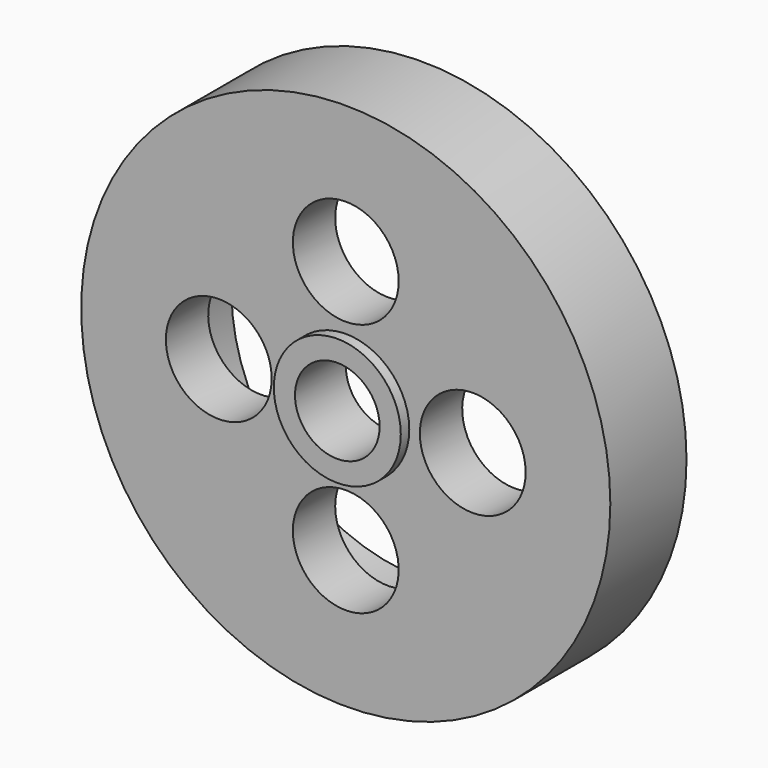
from build123d import *

# Parameters (mm, degrees)
F0_R            = 25
F0_R_2          = 18
F0_R_3          = 6
F0_R_4          = 5
F0_R_5          = 4
F1_DEPTH        = 9
F2_DEPTH        = 10
F3_DEPTH        = 4
F4_DEPTH        = 10.001
F4_COPIES_COUNT = 4


# Not quite as in the source:
# - a pattern or mirror of a feature is missing from the dataset's text; its kind, count and spacing are read off the source's solid


with BuildPart() as f1:
    # F0 (on Front) → F1 (new body)
    with BuildSketch(Plane.XZ):
        Circle(F0_R)
        Circle(F0_R_2, mode=Mode.SUBTRACT)
        Circle(F0_R_2)
        Circle(F0_R_3, mode=Mode.SUBTRACT)
        with Locations((0, 12)):
            Circle(F0_R_4, mode=Mode.SUBTRACT)
        Circle(F0_R_3)
        Circle(F0_R_5, mode=Mode.SUBTRACT)
        with Locations((0, 12)):
            Circle(F0_R_4)
    extrude(amount=F1_DEPTH)

    # F0 (on Front) → F2 (join)
    with BuildSketch(Plane.XZ):
        Circle(F0_R_3)
        Circle(F0_R_5, mode=Mode.SUBTRACT)
    extrude(amount=F2_DEPTH)

    # F0 (on Front) → F3 (cut)
    with BuildSketch(Plane.XZ):
        Circle(F0_R_2)
        Circle(F0_R_3, mode=Mode.SUBTRACT)
        with Locations((0, 12)):
            Circle(F0_R_4, mode=Mode.SUBTRACT)
        Circle(F0_R_3)
        Circle(F0_R_5, mode=Mode.SUBTRACT)
        with Locations((0, 12)):
            Circle(F0_R_4)
    extrude(amount=F3_DEPTH, mode=Mode.SUBTRACT)

    # F0 (on Front) → F4 (cut, through all)
    with BuildSketch(Plane.XZ):
        with Locations((0, 12)):
            Circle(F0_R_4)
    f4 = extrude(amount=F4_DEPTH, mode=Mode.SUBTRACT)

    # F4_copies: F4 ×4 about axis
    f4_copies_axis = Axis((0, 0, 0), (0, 1, 0))
    for i in range(1, F4_COPIES_COUNT):
        add(f4.rotate(f4_copies_axis, i * 360 / F4_COPIES_COUNT), mode=Mode.SUBTRACT)


solid = f1.part
